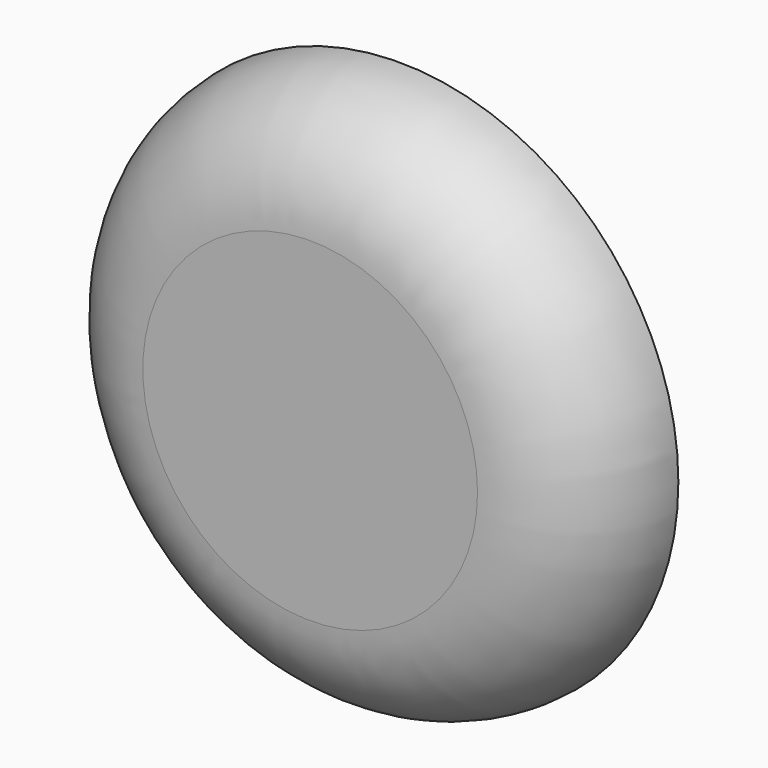
from build123d import *

# Parameters (mm, degrees)
F0_R     = 63.5
F1_DEPTH = 25.4
F2_R     = 25.39999


# Not quite as in the source:
# - a fillet or chamfer is up to 0.001 mm smaller than in the source, because OpenCascade refuses the exact size


with BuildPart() as f1:
    # F0 (on Front) → F1 (new body)
    with BuildSketch(Plane.XZ):
        Circle(F0_R)
    extrude(amount=F1_DEPTH)

    # F2 (radius 25.4 in the source; OpenCascade refuses exactly that, so slightly less here)
    f2_edges = [f1.edges().sort_by_distance(p)[0] for p in [
        (-63.5, -25.4, 0),
    ]]
    fillet(f2_edges, radius=F2_R)


solid = f1.part
